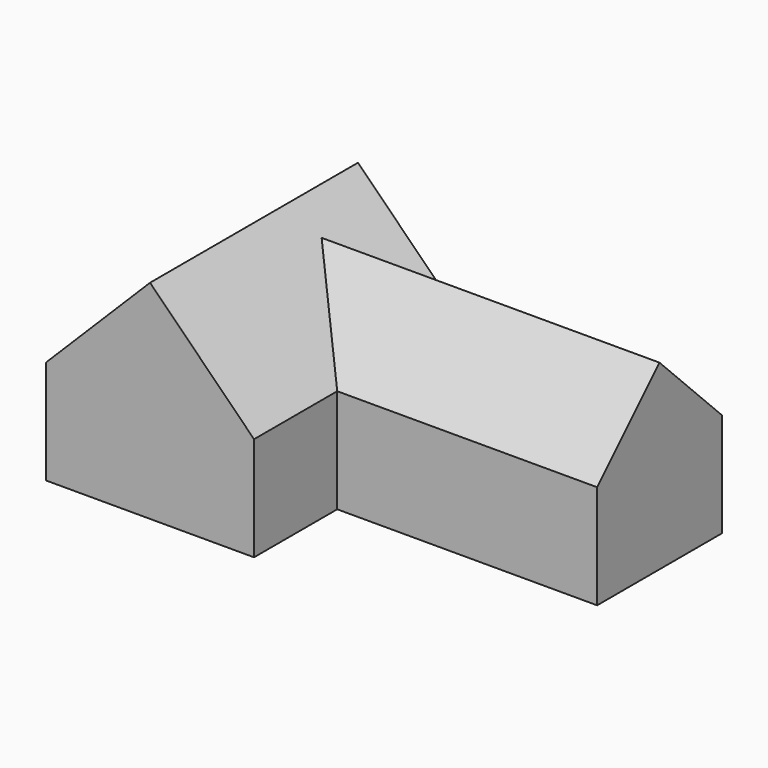
from build123d import *

# Parameters (mm, degrees)
F1_DEPTH = 25.4
F0_W     = 31.75
F0_H     = 19.05
F2_DEPTH = 22.225
F3_SIZE  = 12.69999
F4_SIZE  = 9.52499


# Not quite as in the source:
# - a fillet or chamfer is up to 0.001 mm smaller than in the source, because OpenCascade refuses the exact size


with BuildPart() as f1:
    # F0 (on Top) → F1 (new body)
    with BuildSketch(Plane.XY):
        Polygon((0, 31.75), (0, 0), (25.4, 0), (25.4, 12.7), (25.4, 31.75), align=None)
    extrude(amount=F1_DEPTH)

    # F0 (on Top) → F2 (join)
    with BuildSketch(Plane.XY):
        Polygon((0, 31.75), (0, 0), (25.4, 0), (25.4, 12.7), (25.4, 31.75), align=None)
        with Locations((41.275, 22.225)):
            Rectangle(F0_W, F0_H)
    extrude(amount=F2_DEPTH)

    # F3 (size 12.7 in the source; OpenCascade refuses exactly that, so slightly less here)
    f3_edges = [f1.edges().sort_by_distance(p)[0] for p in [
        (25.4, 15.875, 25.4),
        (0, 15.875, 25.4),
    ]]
    chamfer(f3_edges, length=F3_SIZE)

    # F4 (size 9.525 in the source; OpenCascade refuses exactly that, so slightly less here)
    f4_edges = [f1.edges().sort_by_distance(p)[0] for p in [
        (36.512505, 12.7, 22.225),
        (36.512505, 31.75, 22.225),
    ]]
    chamfer(f4_edges, length=F4_SIZE)


solid = f1.part
